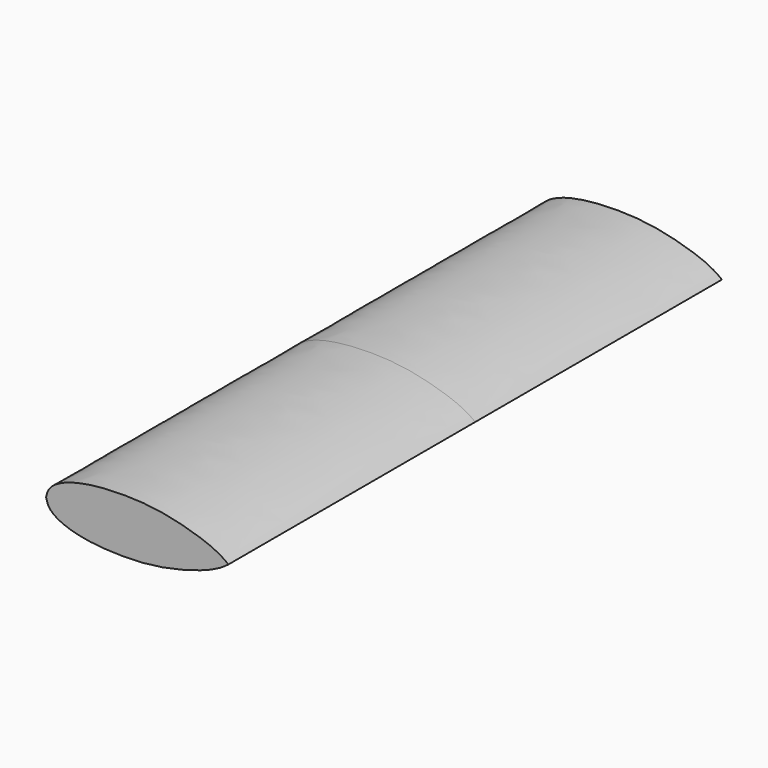
from build123d import *

# Parameters (mm, degrees)
F1_DEPTH      = 254
F1_DEPTH_BACK = 254


with BuildPart() as f1:
    # F0 (on Front) → F1 (new body, two sides)
    with BuildSketch(Plane.XZ) as f1_sk:
        with BuildLine():
            add(Edge.make_bspline(
                [(0, 0), (0.6286497509, 2.6552953814), (2.3559909202, 9.671491677), (25.0945502442, 21.1681196487), (73.8355974202, 23.7133043543), (108.9957265805, 17.9376394921), (138.7762257202, 8.253001806), (147.0530470452, 2.3922072484), (150.2190083265, 0)],
                knots=[0, 0, 0, 0, 0.0972783885, 0.2570931753, 0.491137198, 0.6957410328, 0.8783380364, 1, 1, 1, 1], degree=3))
            Line((0, 0), (150.2190083265, 0))
        make_face()
    extrude(amount=F1_DEPTH)
    extrude(f1_sk.sketch, amount=-F1_DEPTH_BACK)

    # F2: F1 across face


with BuildPart() as f1_1:
    add(f1.part)
    add(f1.part.mirror(Plane(origin=(75.1095041633, 0, 0), x_dir=(1, 0, 0), z_dir=(0, 0, -1))))


solid = f1_1.part
